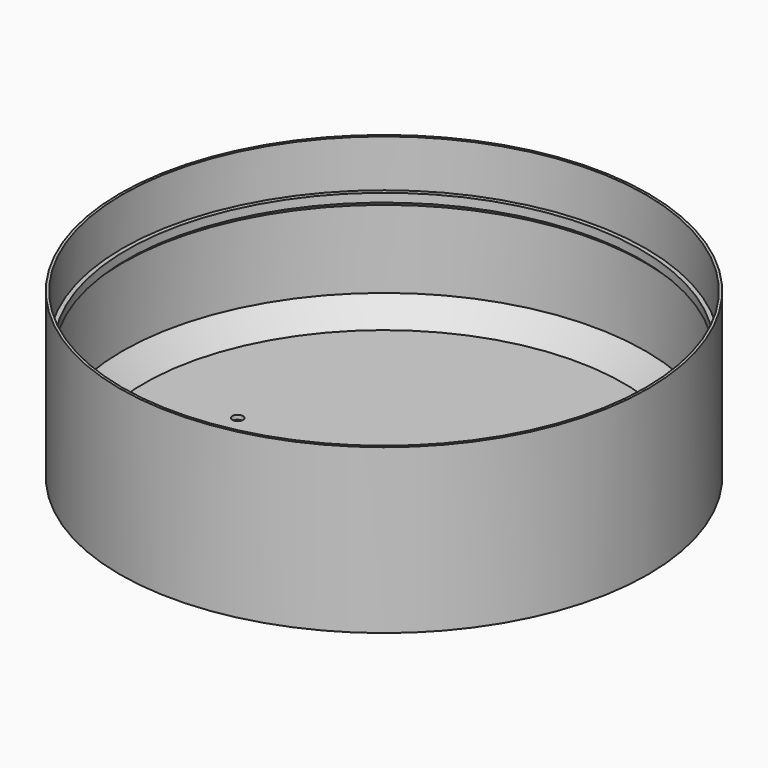
from build123d import *

# Parameters (mm, degrees)
F0_R        = 61.35
F0_R_2      = 1.25
F0_R_3      = 5.5
F1_DEPTH    = 2
F2_R        = 61.35
F2_R_2      = 60.75
F3_DEPTH    = 37
F2_R_3      = 59.75
F4_DEPTH    = 26
F5_DEPTH    = 25
F6_S5_R     = 59.75
F6_T6_DEPTH = 87
F7_SIZE     = 5
F8_DEPTH    = 1


# Not quite as in the source:
# - a fillet or chamfer that OpenCascade refuses, or shapes differently, is made with other operations: its cross-section is extruded or revolved along the edge and cut away or added


with BuildPart() as f1:
    # F0 (on Top) → F1 (new body)
    with BuildSketch(Plane.XY):
        Circle(F0_R)
        with Locations((17, -29.4448637287)):
            Circle(F0_R_2, mode=Mode.SUBTRACT)
        with Locations((-34, 0)):
            Circle(F0_R_2, mode=Mode.SUBTRACT)
        Circle(F0_R_3, mode=Mode.SUBTRACT)
        with Locations((17, 29.4448637287)):
            Circle(F0_R_2, mode=Mode.SUBTRACT)
    extrude(amount=F1_DEPTH)

    # F2 (on face) → F3 (join)
    with BuildSketch(Plane.XY.offset(2)):
        Circle(F2_R)
        Circle(F2_R_2, mode=Mode.SUBTRACT)
    extrude(amount=F3_DEPTH)

    # F2 (on face) → F4 (join)
    with BuildSketch(Plane.XY.offset(2)):
        Circle(F2_R_2)
        Circle(F2_R_3, mode=Mode.SUBTRACT)
    extrude(amount=F4_DEPTH)

    # F2 (on face) → F5 (cut)
    with BuildSketch(Plane.XY.offset(2)):
        Circle(F2_R_2)
        Circle(F2_R_3, mode=Mode.SUBTRACT)
    extrude(amount=F5_DEPTH, mode=Mode.SUBTRACT)

    # F6: chamfer of 2 on 1 edges, made by hand


with BuildPart() as f6_tool2:
    # F6_s3 → F6_t4 (revolve)
    with BuildSketch(Plane.XZ):
        Polygon((60.75, 25), (58.75, 27), (60.75, 27), align=None)
    revolve(axis=Axis((0, 0, 27), (0, 0, 1)))

    # F6_s5 → F6_t6 (cut, symmetric)
    with BuildSketch(Plane.XY.offset(26)):
        Circle(F6_S5_R)
    extrude(amount=F6_T6_DEPTH, both=True, mode=Mode.SUBTRACT)


with BuildPart() as f1_1:
    add(f1.part)

    # F6_t1: union F6_tool2
    add(f6_tool2.part)

    # F7
    f7_edges = [f1_1.edges().sort_by_distance(p)[0] for p in [
        (-60.75, 0, 2),
    ]]
    chamfer(f7_edges, length=F7_SIZE)

    # F8 (cut): a face of the model
    f8_faces = [f1_1.faces().sort_by_distance(p)[0] for p in [
        (-59.614759959, 0, 0),
    ]]
    extrude(f8_faces, amount=-F8_DEPTH, mode=Mode.SUBTRACT)


solid = f1_1.part
